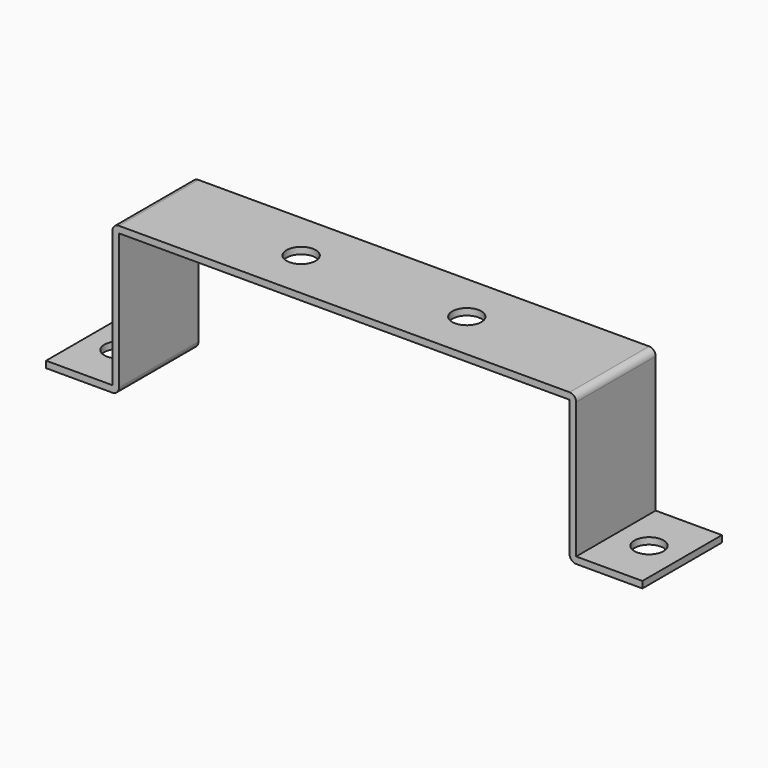
from build123d import *

# Parameters (mm, degrees)
F1_DEPTH = 30
F2_R     = 4.4
F3_R     = 4.4
F4_DEPTH = 25
F5_R     = 2
F6_R     = 2


# Not quite as in the source:
# - a feature names something its author has since deleted; it is built from what else it names


with BuildPart() as f1:
    # F0 (on Front) → F1 (new body)
    with BuildSketch(Plane.XZ):
        Polygon((90, -1), (90, 1), (70, 1), (70, 44), (-70, 44), (-70, 1), (-90, 1), (-90, -1), (-68, -1), (-68, 42), (68, 42), (68, -1), align=None)
    extrude(amount=F1_DEPTH)

    # F2 (on face) + F3 (on face) → F4 (cut)
    with BuildSketch(Plane.XY.offset(1)):
        with Locations((-80, -15)):
            Circle(F2_R)
        with Locations((80, -15)):
            Circle(F2_R)
    with BuildSketch(Plane.XY.offset(44)):
        with Locations((-25, -15)):
            Circle(F3_R)
        with Locations((25, -15)):
            Circle(F3_R)
    extrude(amount=-F4_DEPTH, mode=Mode.SUBTRACT)

    # F5
    f5_edges = [f1.edges().sort_by_distance(p)[0] for p in [
        (-70, -15, 44),
        (70, -15, 44),
    ]]
    fillet(f5_edges, radius=F5_R)

    # F6
    f6_edges = [f1.edges().sort_by_distance(p)[0] for p in [
        (68, -15, -1),
        (-68, -15, -1),
    ]]
    fillet(f6_edges, radius=F6_R)


solid = f1.part
